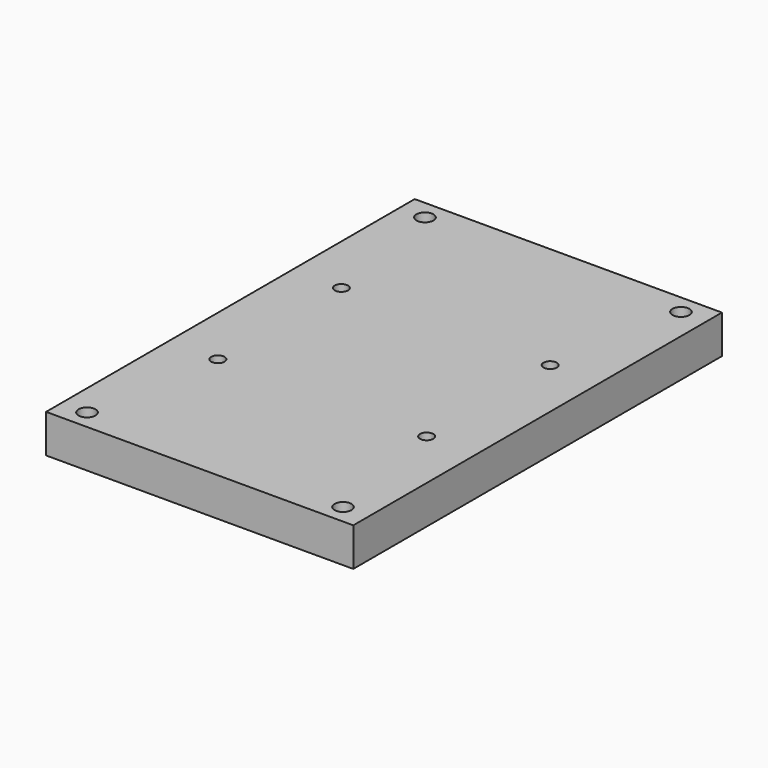
from build123d import *

# Parameters (mm, degrees)
F0_W     = 76.2
F0_H     = 114.3
F1_DEPTH = 9.525
F3_D     = 4.2
F6_D     = 3.3
F6_DEPTH = 12
F6_TIP   = 0.9914200214


# Not quite as in the source:
# - a pattern or mirror of a feature is missing from the dataset's text; its kind, count and spacing are read off the source's solid
# - a feature names something its author has since deleted; it is built from what else it names


with BuildPart() as f1:
    # F0 (on Top) → F1 (new body)
    with BuildSketch(Plane.XY):
        Rectangle(F0_W, F0_H)
    extrude(amount=F1_DEPTH)

    # F3 (through all)
    with Locations(Plane.XY.offset(9.525)):
        with Locations((-31.75, 52.3875), (31.75, 52.3875), (31.75, -52.3875), (-31.75, -52.3875)):
            Hole(F3_D / 2)

    # F6
    with Locations(Plane.XY.offset(9.525)):
        with Locations((-25.9, -19.15), (25.9, -19.15)):
            f6 = Hole(F6_D / 2, depth=F6_DEPTH)
            with Locations((0, 0, -(F6_DEPTH + F6_TIP / 2))):  # 118° drill point
                Cone(0, F6_D / 2, F6_TIP, mode=Mode.SUBTRACT)

    # F6_copies: F6 across plane
    add(f6.mirror(Plane.ZX), mode=Mode.SUBTRACT)


solid = f1.part
